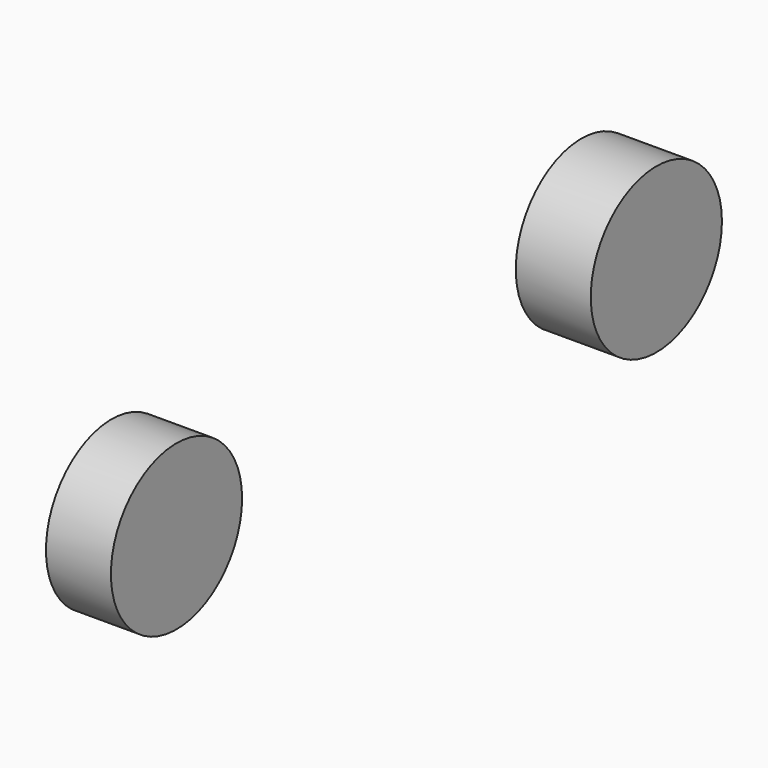
from build123d import *

# Parameters (mm, degrees)
F6_R     = 328
F6_R_2   = 254
F7_DEPTH = 260
F8_DEPTH = 300


# Not quite as in the source:
# - the program builds the solid bodies; features that only make, move or delete a surface that nothing else refers to are left out


with BuildPart() as f7:
    # F6 (on offset) → F7 (new body)
    with BuildSketch(Plane.YZ.offset(637.5)):
        with Locations((-865.8564463551, -88.1656349745)):
            Circle(F6_R)
        with Locations((-865.8564463551, -88.1656349745)):
            Circle(F6_R_2, mode=Mode.SUBTRACT)
        with Locations((-865.8564463551, -88.1656349745)):
            Circle(F6_R_2)
    extrude(amount=-F7_DEPTH)


with BuildPart() as f8:
    # F6 (on offset) → F8 (new body)
    with BuildSketch(Plane.YZ.offset(637.5)):
        with Locations((1534.1435536449, -88.1656349745)):
            Circle(F6_R)
        with Locations((1534.1435536449, -88.1656349745)):
            Circle(F6_R_2, mode=Mode.SUBTRACT)
        with Locations((1534.1435536449, -88.1656349745)):
            Circle(F6_R_2)
    extrude(amount=-F8_DEPTH)


solid = Compound([f7.part, f8.part])
